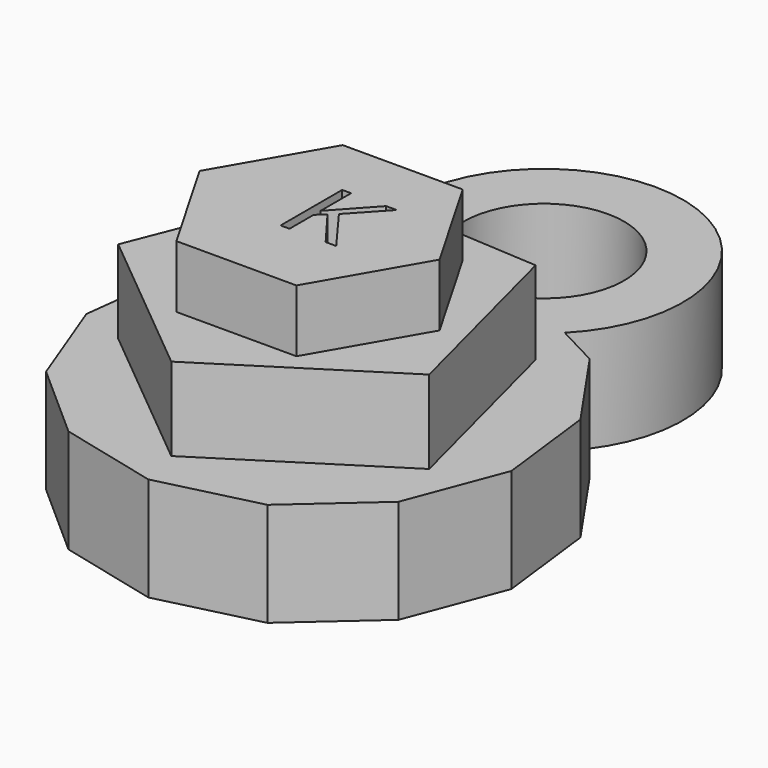
from build123d import *

# Parameters (mm, degrees)
F1_DEPTH     = 6.35
F3_DEPTH     = 5.08
F5_DEPTH     = 3.81
F6_TEXT_SIZE = 6.5921369242
F7_DEPTH     = 6.35
F8_R         = 8.4967167741
F8_R_2       = 4.8972599513
F9_DEPTH     = 6.35


# Not quite as in the source:
# - Text() gives the source's letters only with a copy of the font that has no kerning and outlines rounded to 1/6400 em; it was checked with that copy


with BuildPart() as f1:
    # F0 (on Top) → F1 (new body)
    with BuildSketch(Plane.XY):
        Polygon((3.1302688605, 12.7), (-3.1302688605, 12.7), (-8.6736997094, 9.7905830516), (-12.2300904843, 4.6382615154), (-12.9847149178, -1.5766298369), (-10.7646976464, -7.430334294), (-6.0786178729, -11.5818387096), (0, -13.0800834531), (6.0786178729, -11.5818387096), (10.7646976464, -7.430334294), (12.9847149178, -1.5766298369), (12.2300904843, 4.6382615154), (8.6736997094, 9.7905830516), align=None)
    extrude(amount=F1_DEPTH)

    # F2 (on face) → F3 (join)
    with BuildSketch(Plane.XY.offset(6.35)):
        Polygon((6.7050925159, 8.1200289822), (-5.6506189398, 8.8861488799), (-10.1973670781, -2.6280869453), (-0.6517005103, -10.5103959375), (9.7945940123, -3.8676949793), align=None)
    extrude(amount=F3_DEPTH)

    # F4 (on face) → F5 (join)
    with BuildSketch(Plane.XY.offset(11.43)):
        Polygon((3.6661742094, 6.35), (-3.6661742094, 6.35), (-7.3323484187, 0), (-3.6661742094, -6.35), (3.6661742094, -6.35), (7.3323484187, 0), align=None)
    extrude(amount=F5_DEPTH)

    # F6 (on face) → F7 (cut)
    with BuildSketch(Plane.XY.offset(15.24)):
        with Locations((-1.4423821121, -1.983087277)):
            Text('K', F6_TEXT_SIZE, font='Open Sans', text_align=(TextAlign.LEFT, TextAlign.BOTTOM))
    extrude(amount=-F7_DEPTH, mode=Mode.SUBTRACT)

    # F8 (on Top) → F9 (join, through all)
    with BuildSketch(Plane.XY):
        with Locations((0, 17.1357635409)):
            Circle(F8_R)
        with Locations((0, 17.1357635409)):
            Circle(F8_R_2, mode=Mode.SUBTRACT)
    extrude(amount=F9_DEPTH)


solid = f1.part
